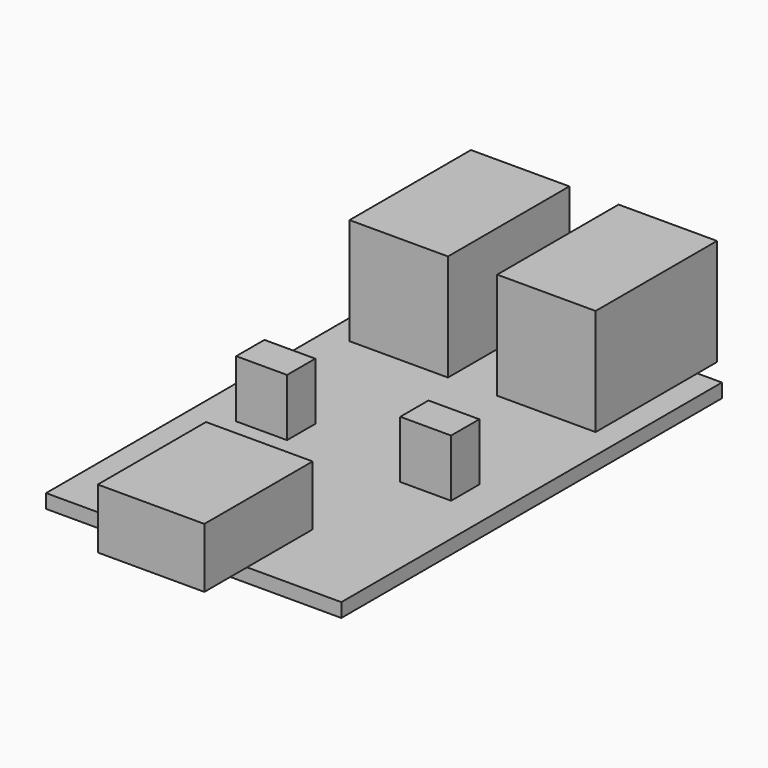
from build123d import *

# Parameters (mm, degrees)
F0_W     = 6.2
F0_H     = 4.3
F0_W_2   = 12
F0_H_2   = 15.5
F0_W_3   = 13
F0_H_3   = 10
F1_DEPTH = 1.7
F0_H_4   = 6.5
F2_DEPTH = 7.3
F0_H_5   = 3
F3_DEPTH = 13
F4_DEPTH = 7


with BuildPart() as f1:
    # F0 (on Top) → F1 (new body)
    with BuildSketch(Plane.XY):
        Polygon((18, -29), (18, 29), (15, 29), (15, 13.5), (3, 13.5), (3, 29), (-3, 29), (-3, 13.5), (-15, 13.5), (-15, 29), (-18, 29), (-18, -29), (-6.5, -29), (-6.5, -19), (6.5, -19), (6.5, -29), align=None)
        with Locations((-10, -4)):
            Rectangle(F0_W, F0_H, mode=Mode.SUBTRACT)
        with Locations((10, -4)):
            Rectangle(F0_W, F0_H, mode=Mode.SUBTRACT)
        with Locations((9, 21.25)):
            Rectangle(F0_W_2, F0_H_2)
        with Locations((-9, 21.25)):
            Rectangle(F0_W_2, F0_H_2)
        with Locations((0, -24)):
            Rectangle(F0_W_3, F0_H_3)
        with Locations((10, -4)):
            Rectangle(F0_W, F0_H)
        with Locations((-10, -4)):
            Rectangle(F0_W, F0_H)
    extrude(amount=-F1_DEPTH)


with BuildPart() as f2:
    # F0 (on Top) → F2 (new body)
    with BuildSketch(Plane.XY):
        with Locations((0, -32.25)):
            Rectangle(F0_W_3, F0_H_4)
        with Locations((0, -24)):
            Rectangle(F0_W_3, F0_H_3)
    extrude(amount=F2_DEPTH)


with BuildPart() as f3:
    # F0 (on Top) → F3 (new body)
    with BuildSketch(Plane.XY):
        with Locations((-9, 30.5)):
            Rectangle(F0_W_2, F0_H_5)
        with Locations((-9, 21.25)):
            Rectangle(F0_W_2, F0_H_2)
    extrude(amount=F3_DEPTH)


with BuildPart() as f3b:
    # F0 (on Top) → F3, piece 2 (new body)
    with BuildSketch(Plane.XY):
        with Locations((9, 21.25)):
            Rectangle(F0_W_2, F0_H_2)
        with Locations((9, 30.5)):
            Rectangle(F0_W_2, F0_H_5)
    extrude(amount=F3_DEPTH)


with BuildPart() as f4:
    # F0 (on Top) → F4 (new body)
    with BuildSketch(Plane.XY):
        with Locations((10, -4)):
            Rectangle(F0_W, F0_H)
    extrude(amount=F4_DEPTH)


with BuildPart() as f4b:
    # F0 (on Top) → F4, piece 2 (new body)
    with BuildSketch(Plane.XY):
        with Locations((-10, -4)):
            Rectangle(F0_W, F0_H)
    extrude(amount=F4_DEPTH)


solid = Compound([f1.part, f2.part, f3.part, f3b.part, f4.part, f4b.part])
